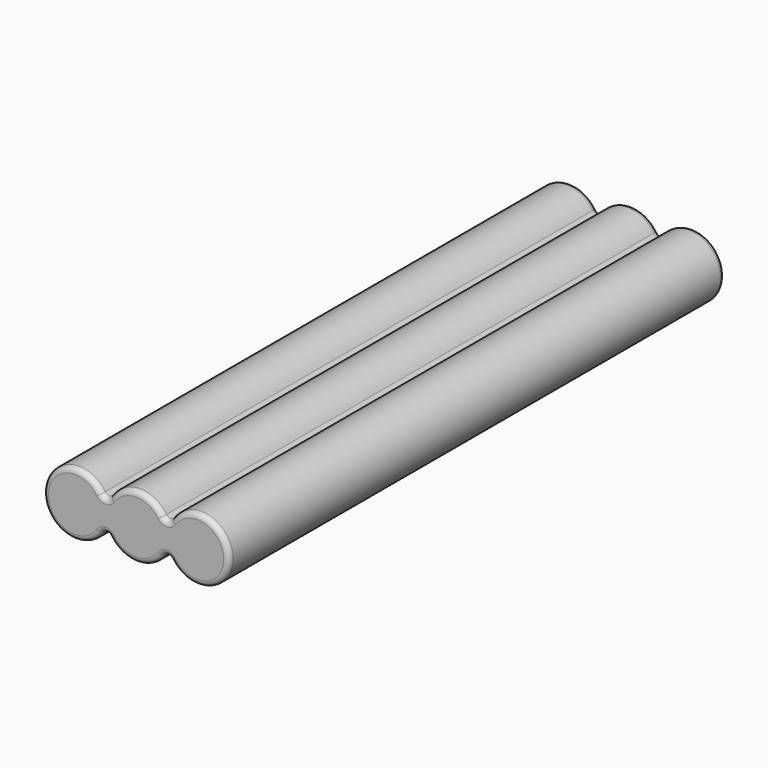
from build123d import *

# Parameters (mm, degrees)
F1_DEPTH = 74.6125
F2_R     = 1.27


with BuildPart() as f1:
    # F0 (on Front) → F1 (new body, symmetric)
    with BuildSketch(Plane.XZ):
        with BuildLine():
            ThreePointArc((-7.3719540369, 1.9283914741), (-22.3639080738, 0), (-7.3719540369, -1.9283914741))
            ThreePointArc((-7.3719540369, -1.9283914741), (0, -7.62), (7.3719540369, -1.9283914741))
            ThreePointArc((7.3719540369, -1.9283914741), (22.3639080738, 0), (7.3719540369, 1.9283914741))
            ThreePointArc((7.3719540369, 1.9283914741), (0, 7.62), (-7.3719540369, 1.9283914741))
        make_face()
    extrude(amount=F1_DEPTH, both=True)

    # F2
    f2_edges = [f1.edges().sort_by_distance(p)[0] for p in [
        (7.371954, 0, 1.928391),
        (0, 74.6125, 7.62),
        (-7.371954, 0, 1.928391),
        (0, -74.6125, 7.62),
        (7.371954, 0, -1.928391),
        (22.363908, 74.6125, 0),
        (22.363908, -74.6125, 0),
        (-22.363908, 74.6125, 0),
        (-7.371954, 0, -1.928391),
        (-22.363908, -74.6125, 0),
        (0, 74.6125, -7.62),
        (0, -74.6125, -7.62),
    ]]
    fillet(f2_edges, radius=F2_R)


solid = f1.part
